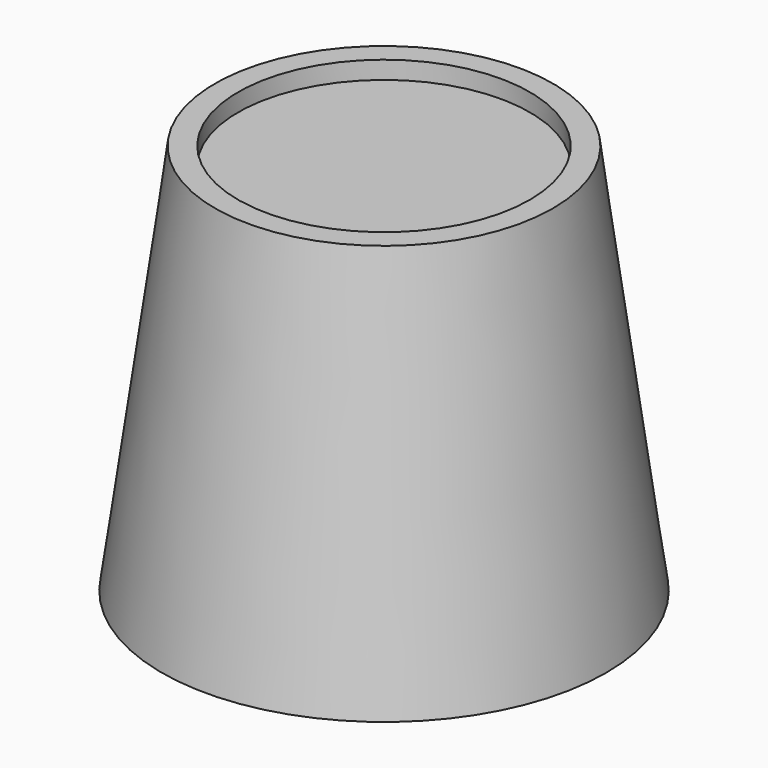
from build123d import *

# Parameters (mm, degrees)
F0_R     = 62.5
F1_DEPTH = 110
F2_SIZE2 = 109.99999
F2_SIZE  = 14.99999
F3_R     = 41
F4_DEPTH = 5


# Not quite as in the source:
# - a fillet or chamfer is up to 0.001 mm smaller than in the source, because OpenCascade refuses the exact size


with BuildPart() as f1:
    # F0 (on Top) → F1 (new body)
    with BuildSketch(Plane.XY):
        Circle(F0_R)
    extrude(amount=F1_DEPTH)

    # F2 (size 15 and 110 in the source; OpenCascade refuses exactly that, so slightly less here)
    f2_edges = [f1.edges().sort_by_distance(p)[0] for p in [
        (-62.5, 0, 110),
    ]]
    f2_side = f1.faces().sort_by_distance((0, 0, 110))[0]
    chamfer(f2_edges, length=F2_SIZE, length2=F2_SIZE2, reference=f2_side)

    # F3 (on face) → F4 (cut)
    with BuildSketch(Plane.XY.offset(110)):
        Circle(F3_R)
    extrude(amount=-F4_DEPTH, mode=Mode.SUBTRACT)


solid = f1.part
